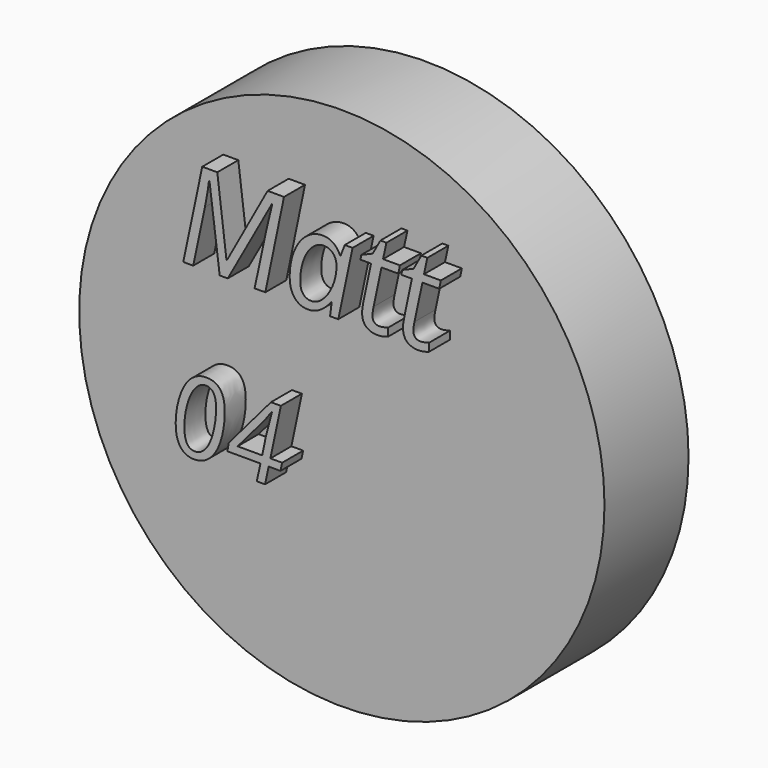
from build123d import *

# Parameters (mm, degrees)
F0_R           = 63.5
F1_DEPTH       = 25.4
F2_TEXT_SIZE   = 30.4988714763
F2_TEXT_SIZE_2 = 25.0114852356
F3_DEPTH       = 6.35


# Not quite as in the source:
# - Text() gives the source's letters only with a copy of the font that has no kerning and outlines rounded to 1/6400 em; it was checked with that copy


with BuildPart() as f1:
    # F0 (on Front) → F1 (new body)
    with BuildSketch(Plane.XZ):
        Circle(F0_R)
    extrude(amount=F1_DEPTH)

    # F2 (on face) → F3 (join)
    with BuildSketch(Plane.XZ.offset(25.4)):
        with Locations((-34.5193445683, 22.886922583)):
            Text('Matt', F2_TEXT_SIZE, font='Open Sans', font_style=FontStyle.ITALIC, text_align=(TextAlign.LEFT, TextAlign.BOTTOM))
        with Locations((-36.5686826408, -18.0082693696)):
            Text('04', F2_TEXT_SIZE_2, font='Open Sans', font_style=FontStyle.ITALIC, text_align=(TextAlign.LEFT, TextAlign.BOTTOM))
    extrude(amount=F3_DEPTH)


solid = f1.part
